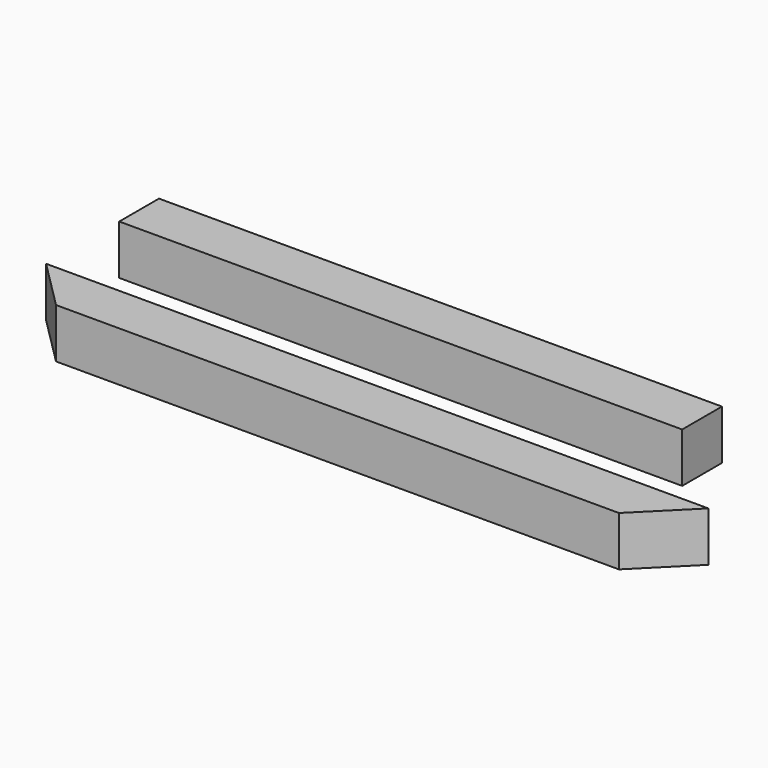
from build123d import *

# Parameters (mm, degrees)
F0_W     = 1200
F0_H     = 90
F1_DEPTH = 90
F2_SIZE  = 89.99999
F3_W     = 1020
F3_H     = 90
F4_DEPTH = 90


# Not quite as in the source:
# - a fillet or chamfer is up to 0.001 mm smaller than in the source, because OpenCascade refuses the exact size


with BuildPart() as f1:
    # F0 (on Top) → F1 (new body)
    with BuildSketch(Plane.XY):
        with Locations((600, -45)):
            Rectangle(F0_W, F0_H)
    extrude(amount=F1_DEPTH)

    # F2 (size 90 in the source; OpenCascade refuses exactly that, so slightly less here)
    f2_edges = [f1.edges().sort_by_distance(p)[0] for p in [
        (1200, -90, 45),
        (0, -90, 45),
    ]]
    chamfer(f2_edges, length=F2_SIZE)


with BuildPart() as f4:
    # F3 (on Top) → F4 (new body)
    with BuildSketch(Plane.XY):
        with Locations((510, 210.6959205866)):
            Rectangle(F3_W, F3_H)
    extrude(amount=F4_DEPTH)


solid = Compound([f1.part, f4.part])
